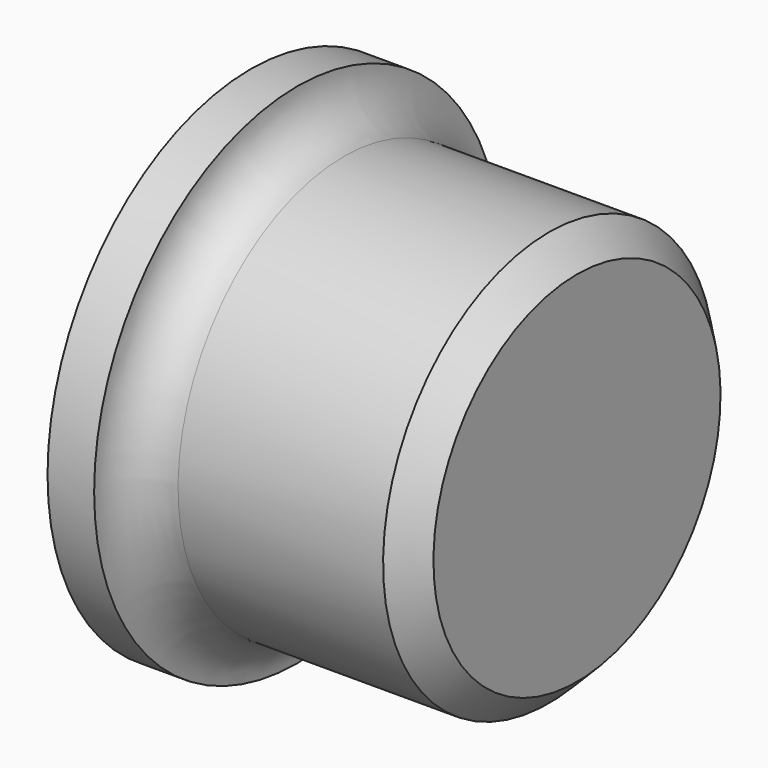
from build123d import *

# Parameters (mm, degrees)
F2_SIZE = 3
F3_R    = 4.99999


# Not quite as in the source:
# - a fillet or chamfer is up to 0.001 mm smaller than in the source, because OpenCascade refuses the exact size


with BuildPart() as f1:
    # F0 (on Front) → F1 (revolve)
    with BuildSketch(Plane.XZ):
        Polygon((-64, 22.25), (-94, 22.25), (-94, 27.25), (-99, 27.25), (-99, 0), (-64, 0), align=None)
    revolve(axis=Axis((-47, 0, 0), (-1, 0, 0)))

    # F2
    f2_edges = [f1.edges().sort_by_distance(p)[0] for p in [
        (-64, 0, -22.25),
    ]]
    chamfer(f2_edges, length=F2_SIZE)

    # F3 (radius 5 in the source; OpenCascade refuses exactly that, so slightly less here)
    f3_edges = [f1.edges().sort_by_distance(p)[0] for p in [
        (-94, 0, -22.25),
    ]]
    fillet(f3_edges, radius=F3_R)


solid = f1.part
